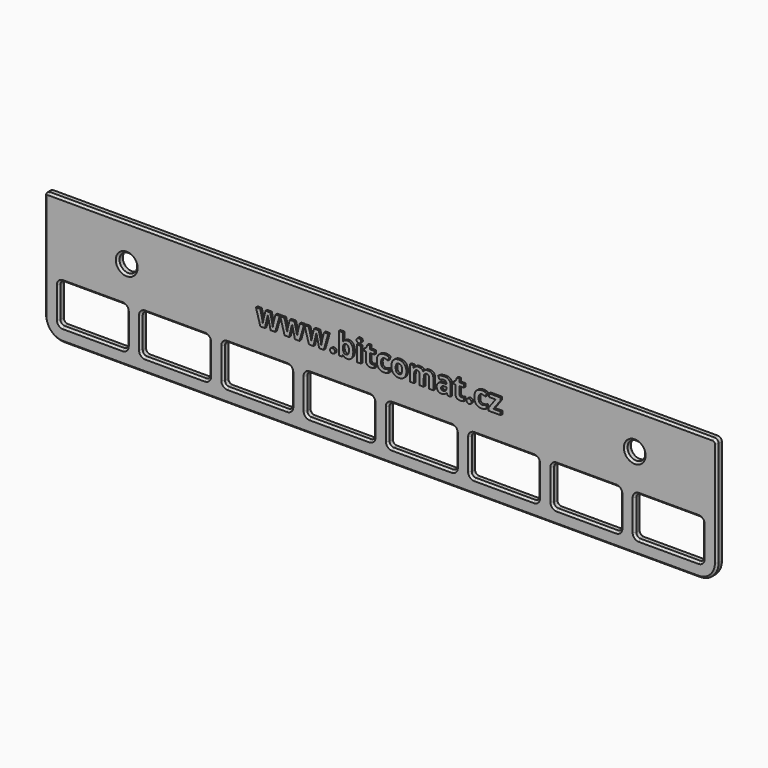
from build123d import *

# Parameters (mm, degrees)
F0_W         = 163.5
F0_H         = 31
F0_W_2       = 16.5
F0_H_2       = 9.5
F0_R         = 2.15
F1_DEPTH     = 2
F2_R         = 1
F3_R         = 4.5
F4_R         = 1
F5_SIZE      = 0.5
F6_TEXT_SIZE = 6.8960563178
F7_DEPTH     = 0.5


# Not quite as in the source:
# - a feature names something its author has since deleted; it is built from what else it names
# - Text() gives the source's letters only with a copy of the font that has no kerning and outlines rounded to 1/6400 em; it was checked with that copy


with BuildPart() as f1:
    # F0 (on Front) → F1 (new body)
    with BuildSketch(Plane.XZ):
        with Locations((81.75, 15.5)):
            Rectangle(F0_W, F0_H)
        with Locations((11.75, 8.25)):
            Rectangle(F0_W_2, F0_H_2, mode=Mode.SUBTRACT)
        with Locations((31.75, 8.25)):
            Rectangle(F0_W_2, F0_H_2, mode=Mode.SUBTRACT)
        with Locations((51.75, 8.25)):
            Rectangle(F0_W_2, F0_H_2, mode=Mode.SUBTRACT)
        with Locations((71.75, 8.25)):
            Rectangle(F0_W_2, F0_H_2, mode=Mode.SUBTRACT)
        with Locations((91.75, 8.25)):
            Rectangle(F0_W_2, F0_H_2, mode=Mode.SUBTRACT)
        with Locations((111.75, 8.25)):
            Rectangle(F0_W_2, F0_H_2, mode=Mode.SUBTRACT)
        with Locations((131.75, 8.25)):
            Rectangle(F0_W_2, F0_H_2, mode=Mode.SUBTRACT)
        with Locations((151.75, 8.25)):
            Rectangle(F0_W_2, F0_H_2, mode=Mode.SUBTRACT)
        with Locations((20, 22)):
            Circle(F0_R, mode=Mode.SUBTRACT)
        with Locations((143.5, 22)):
            Circle(F0_R, mode=Mode.SUBTRACT)
    extrude(amount=F1_DEPTH)

    # F2
    f2_edges = [f1.edges().sort_by_distance(p)[0] for p in [
        (0, -1, 31),
        (163.5, -1, 31),
    ]]
    fillet(f2_edges, radius=F2_R)

    # F3
    f3_edges = [f1.edges().sort_by_distance(p)[0] for p in [
        (0, -1, 0),
        (163.5, -1, 0),
    ]]
    fillet(f3_edges, radius=F3_R)

    # F4
    f4_edges = [f1.edges().sort_by_distance(p)[0] for p in [
        (3.5, -1, 13),
        (23.5, -1, 13),
        (43.5, -1, 13),
        (63.5, -1, 13),
        (83.5, -1, 13),
        (103.5, -1, 13),
        (120, -1, 13),
        (100, -1, 13),
        (80, -1, 13),
        (60, -1, 13),
        (40, -1, 13),
        (20, -1, 13),
        (3.5, -1, 3.5),
        (23.5, -1, 3.5),
        (43.5, -1, 3.5),
        (63.5, -1, 3.5),
        (83.5, -1, 3.5),
        (103.5, -1, 3.5),
        (120, -1, 3.5),
        (100, -1, 3.5),
        (80, -1, 3.5),
        (60, -1, 3.5),
        (40, -1, 3.5),
        (20, -1, 3.5),
        (123.5, -1, 13),
        (140, -1, 13),
        (160, -1, 13),
        (143.5, -1, 13),
        (123.5, -1, 3.5),
        (143.5, -1, 3.5),
        (140, -1, 3.5),
        (160, -1, 3.5),
    ]]
    fillet(f4_edges, radius=F4_R)

    # F5
    f5_edges = [f1.edges().sort_by_distance(p)[0] for p in [
        (3.5, -2, 8.25),
        (3.792893, -2, 3.792893),
        (3.792893, -2, 12.707107),
        (11.75, -2, 3.5),
        (11.75, -2, 13),
        (19.707107, -2, 3.792893),
        (19.707107, -2, 12.707107),
        (20, -2, 8.25),
        (0, -2, 17.25),
        (1.318019, -2, 1.318019),
        (0.292893, -2, 30.707107),
        (81.75, -2, 0),
        (81.75, -2, 31),
        (162.181981, -2, 1.318019),
        (163.207107, -2, 30.707107),
        (163.5, -2, 17.25),
        (17.85, -2, 22),
        (141.35, -2, 22),
        (23.5, -2, 8.25),
        (23.792893, -2, 3.792893),
        (23.792893, -2, 12.707107),
        (31.75, -2, 3.5),
        (31.75, -2, 13),
        (39.707107, -2, 3.792893),
        (39.707107, -2, 12.707107),
        (40, -2, 8.25),
        (43.5, -2, 8.25),
        (43.792893, -2, 3.792893),
        (43.792893, -2, 12.707107),
        (51.75, -2, 3.5),
        (51.75, -2, 13),
        (59.707107, -2, 3.792893),
        (59.707107, -2, 12.707107),
        (60, -2, 8.25),
        (63.5, -2, 8.25),
        (63.792893, -2, 3.792893),
        (63.792893, -2, 12.707107),
        (71.75, -2, 3.5),
        (71.75, -2, 13),
        (79.707107, -2, 3.792893),
        (79.707107, -2, 12.707107),
        (80, -2, 8.25),
        (83.5, -2, 8.25),
        (83.792893, -2, 3.792893),
        (83.792893, -2, 12.707107),
        (91.75, -2, 3.5),
        (91.75, -2, 13),
        (99.707107, -2, 3.792893),
        (99.707107, -2, 12.707107),
        (100, -2, 8.25),
        (103.5, -2, 8.25),
        (103.792893, -2, 3.792893),
        (103.792893, -2, 12.707107),
        (111.75, -2, 3.5),
        (111.75, -2, 13),
        (119.707107, -2, 3.792893),
        (119.707107, -2, 12.707107),
        (120, -2, 8.25),
        (123.5, -2, 8.25),
        (123.792893, -2, 3.792893),
        (123.792893, -2, 12.707107),
        (131.75, -2, 3.5),
        (131.75, -2, 13),
        (139.707107, -2, 3.792893),
        (139.707107, -2, 12.707107),
        (140, -2, 8.25),
        (143.5, -2, 8.25),
        (143.792893, -2, 3.792893),
        (143.792893, -2, 12.707107),
        (151.75, -2, 3.5),
        (151.75, -2, 13),
        (159.707107, -2, 3.792893),
        (159.707107, -2, 12.707107),
        (160, -2, 8.25),
        (3.5, 0, 8.25),
        (3.792893, 0, 3.792893),
        (3.792893, 0, 12.707107),
        (11.75, 0, 3.5),
        (11.75, 0, 13),
        (19.707107, 0, 3.792893),
        (19.707107, 0, 12.707107),
        (20, 0, 8.25),
        (0, 0, 17.25),
        (1.318019, 0, 1.318019),
        (0.292893, 0, 30.707107),
        (81.75, 0, 0),
        (81.75, 0, 31),
        (162.181981, 0, 1.318019),
        (163.207107, 0, 30.707107),
        (163.5, 0, 17.25),
        (17.85, 0, 22),
        (141.35, 0, 22),
        (23.5, 0, 8.25),
        (23.792893, 0, 3.792893),
        (23.792893, 0, 12.707107),
        (31.75, 0, 3.5),
        (31.75, 0, 13),
        (39.707107, 0, 3.792893),
        (39.707107, 0, 12.707107),
        (40, 0, 8.25),
        (43.5, 0, 8.25),
        (43.792893, 0, 3.792893),
        (43.792893, 0, 12.707107),
        (51.75, 0, 3.5),
        (51.75, 0, 13),
        (59.707107, 0, 3.792893),
        (59.707107, 0, 12.707107),
        (60, 0, 8.25),
        (63.5, 0, 8.25),
        (63.792893, 0, 3.792893),
        (63.792893, 0, 12.707107),
        (71.75, 0, 3.5),
        (71.75, 0, 13),
        (79.707107, 0, 3.792893),
        (79.707107, 0, 12.707107),
        (80, 0, 8.25),
        (83.5, 0, 8.25),
        (83.792893, 0, 3.792893),
        (83.792893, 0, 12.707107),
        (91.75, 0, 3.5),
        (91.75, 0, 13),
        (99.707107, 0, 3.792893),
        (99.707107, 0, 12.707107),
        (100, 0, 8.25),
        (103.5, 0, 8.25),
        (103.792893, 0, 3.792893),
        (103.792893, 0, 12.707107),
        (111.75, 0, 3.5),
        (111.75, 0, 13),
        (119.707107, 0, 3.792893),
        (119.707107, 0, 12.707107),
        (120, 0, 8.25),
        (123.5, 0, 8.25),
        (123.792893, 0, 3.792893),
        (123.792893, 0, 12.707107),
        (131.75, 0, 3.5),
        (131.75, 0, 13),
        (139.707107, 0, 3.792893),
        (139.707107, 0, 12.707107),
        (140, 0, 8.25),
        (143.5, 0, 8.25),
        (143.792893, 0, 3.792893),
        (143.792893, 0, 12.707107),
        (151.75, 0, 3.5),
        (151.75, 0, 13),
        (159.707107, 0, 3.792893),
        (159.707107, 0, 12.707107),
        (160, 0, 8.25),
    ]]
    chamfer(f5_edges, length=F5_SIZE)

    # F6 (on face) → F7 (join)
    with BuildSketch(Plane.XZ.offset(2)):
        with Locations((51.75, 19.5174197256)):
            Text('www.bitcomat.cz', F6_TEXT_SIZE, font='Open Sans', font_style=FontStyle.BOLD, text_align=(TextAlign.LEFT, TextAlign.BOTTOM))
    extrude(amount=F7_DEPTH)


solid = f1.part
